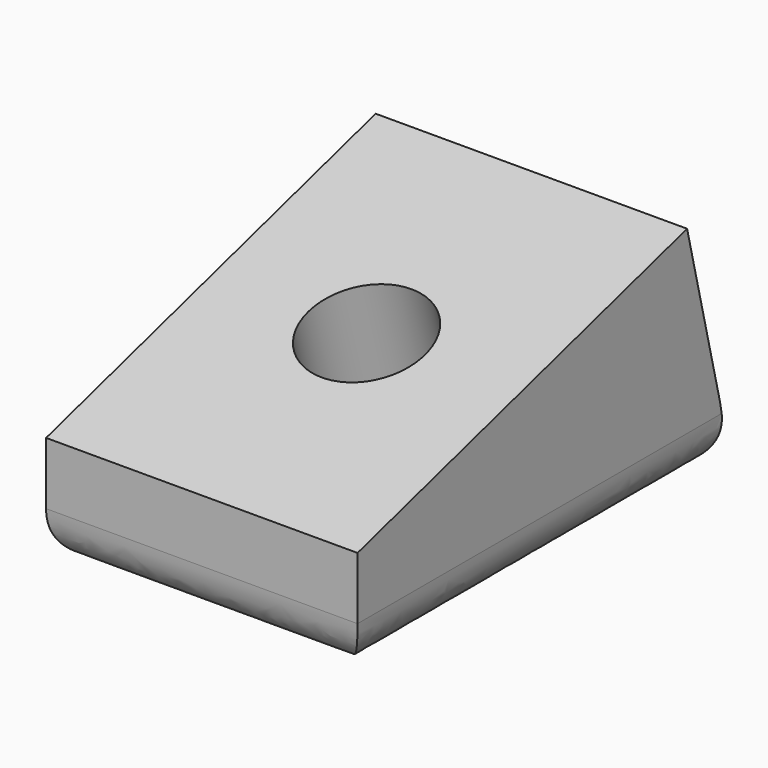
from build123d import *

# Parameters (mm, degrees)
F1_DEPTH    = 25.4
F3_T1_DEPTH = 49.6403917904
F3_T3_DEPTH = 57.15
F3_T5_DEPTH = 44.45
F4_D        = 9.525


# Not quite as in the source:
# - a fillet or chamfer that OpenCascade refuses, or shapes differently, is made with other operations: its cross-section is extruded or revolved along the edge and cut away or added


with BuildPart() as f1:
    # F0 (on Right) → F1 (new body)
    with BuildSketch(Plane.YZ):
        Polygon((28.2472143829, 0), (23.7438723809, 18.5100624206), (-9.8527856171, 8.89), (-9.8527856171, 0), align=None)
    extrude(amount=F1_DEPTH)

    # F3: fillet of radius 3.81 on 4 edges, made by hand

    # F3_s2 → F3_t1 (cut)
    with BuildSketch(Plane.YZ.offset(-12.1201958952)):
        with BuildLine():
            add(Edge.make_bspline(
                [(23.3991360248, 0), (28.2472143829, 0), (27.1011485089, 4.7106684004)],
                knots=[0, 0, 0, 1, 1, 1], degree=2, weights=[1, 1, 1]))
            Line((27.1011485089, 4.7106684004), (28.2472143829, 0))
            Line((28.2472143829, 0), (23.3991360248, 0))
        make_face()
    extrude(amount=F3_T1_DEPTH, mode=Mode.SUBTRACT)

    # F3_s4 → F3_t3 (cut)
    with BuildSketch(Plane.XZ.offset(-37.7722143829)):
        with BuildLine():
            add(Edge.make_bspline(
                [(3.81, 0), (0, 0), (0, 3.81)],
                knots=[0, 0, 0, 1, 1, 1], degree=2, weights=[1, 1, 1]))
            Line((0, 3.81), (0, 0))
            Line((0, 0), (3.81, 0))
        make_face()
        with BuildLine():
            add(Edge.make_bspline(
                [(21.59, 0), (25.4, 0), (25.4, 3.81)],
                knots=[0, 0, 0, 1, 1, 1], degree=2, weights=[1, 1, 1]))
            Line((25.4, 3.81), (25.4, 0))
            Line((25.4, 0), (21.59, 0))
        make_face()
    extrude(amount=F3_T3_DEPTH, mode=Mode.SUBTRACT)

    # F3_s6 → F3_t5 (cut)
    with BuildSketch(Plane.YZ.offset(-9.525)):
        with BuildLine():
            add(Edge.make_bspline(
                [(-9.8527856171, 3.81), (-9.8527856171, 0), (-6.0427856171, 0)],
                knots=[0, 0, 0, 1, 1, 1], degree=2, weights=[1, 1, 1]))
            Line((-6.0427856171, 0), (-9.8527856171, 0))
            Line((-9.8527856171, 0), (-9.8527856171, 3.81))
        make_face()
    extrude(amount=F3_T5_DEPTH, mode=Mode.SUBTRACT)

    # F4 (through all)
    with Locations(Plane(origin=(0, -3.0992844266, 10.8237966001), x_dir=(1, 0, 0), z_dir=(0, -0.2752771, 0.9613649246))):
        with Locations((12.7, 10.448506651)):
            Hole(F4_D / 2)


solid = f1.part
